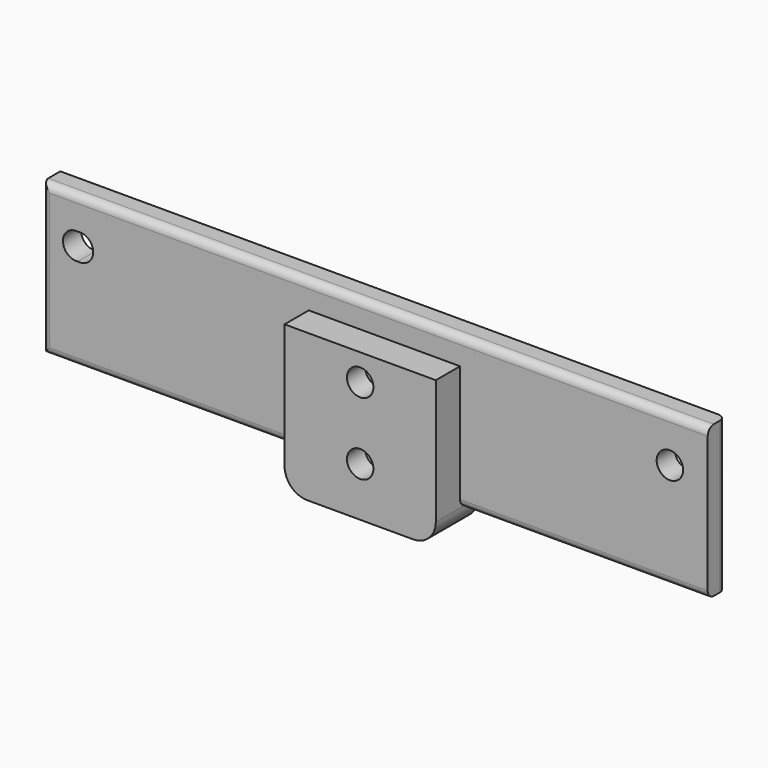
from build123d import *

# Parameters (mm, degrees)
F0_W     = 88
F0_H     = 20
F0_R     = 1.75
F1_DEPTH = 3
F2_W     = 20
F2_H     = 4.5
F2_H_2   = 7.5
F3_DEPTH = 4
F6_DEPTH = 4
F4_R     = 1.75
F7_DEPTH = 25
F9_DEPTH = 3
F10_R    = 3
F11_R    = 1


# Not quite as in the source:
# - a feature names something its author has since deleted; it is built from what else it names


with BuildPart() as f1:
    # F0 (on Front) → F1 (new body)
    with BuildSketch(Plane.XZ):
        with Locations((44, -10)):
            Rectangle(F0_W, F0_H)
        with BuildLine():
            ThreePointArc((35.25, -15.5), (34.0207943633, -16.7498270258), (32.7506918489, -15.5415829716))
            ThreePointArc((32.7506918489, -15.5415829716), (32.75, -15.5), (32.7506918489, -15.4584170284))
            Line((32.7506918489, -15.4584170284), (32.7506918489, -8.0415829716))
            ThreePointArc((32.7506918489, -8.0415829716), (32.75, -8), (32.7506918489, -7.9584170284))
            ThreePointArc((32.7506918489, -7.9584170284), (34.0207943633, -6.7501729742), (35.25, -8))
            Line((35.25, -8), (35.25, -15.5))
        make_face(mode=Mode.SUBTRACT)
        with BuildLine():
            ThreePointArc((4.75, -4.2679491924), (6.1456439237, -4.6771243445), (6.75, -6))
            ThreePointArc((6.75, -6), (6.1456439237, -7.3228756555), (4.75, -7.7320508076))
            ThreePointArc((4.75, -7.7320508076), (2.75, -6), (4.75, -4.2679491924))
        make_face(mode=Mode.SUBTRACT)
        with Locations((83, -6)):
            Circle(F0_R, mode=Mode.SUBTRACT)
    extrude(amount=F1_DEPTH)

    # F2 (on face) → F3 (join)
    with BuildSketch(Plane.XZ.offset(3)):
        with Locations((45.25, -5.75)):
            Rectangle(F2_W, F2_H)
        with Locations((45.25, -11.75)):
            Rectangle(F2_W, F2_H_2)
        with Locations((45.25, -17.75)):
            Rectangle(F2_W, F2_H)
    extrude(amount=F3_DEPTH)

    # F5 (on face) → F6 (cut)
    with BuildSketch(Plane(origin=(0, 0, 0), x_dir=(-1, 0, 0), z_dir=(0, 1, 0))):
        Polygon((-43.5179491924, -4), (-46.9820508076, -4), (-48.7141016151, -7), (-46.9820508076, -10), (-43.5179491924, -10), (-41.7858983849, -7), align=None)
        Polygon((-43.5179491924, -13.5), (-46.9820508076, -13.5), (-48.7141016151, -16.5), (-46.9820508076, -19.5), (-43.5179491924, -19.5), (-41.7858983849, -16.5), align=None)
    extrude(amount=-F6_DEPTH, mode=Mode.SUBTRACT)

    # F4 (on face) → F7 (cut)
    with BuildSketch(Plane.XZ.offset(7)):
        with Locations((45.25, -7)):
            Circle(F4_R)
        with Locations((45.25, -16.5)):
            Circle(F4_R)
    extrude(amount=-F7_DEPTH, mode=Mode.SUBTRACT)

    # F8 (on face) → F9 (join)
    with BuildSketch(Plane(origin=(0, 0, -20), x_dir=(1, 0, 0), z_dir=(0, 0, -1))):
        Polygon((55.25, 3), (55.25, 7), (35.25, 7), (35.25, 3), (35.25, 0), (55.25, 0), align=None)
    extrude(amount=F9_DEPTH)

    # F10
    f10_edges = [f1.edges().sort_by_distance(p)[0] for p in [
        (35.25, -3.5, -23),
        (55.25, -3.5, -23),
    ]]
    fillet(f10_edges, radius=F10_R)

    # F11
    f11_edges = [f1.edges().sort_by_distance(p)[0] for p in [
        (44, -3, 0),
        (88, 0, -10),
        (71.625, -3, -20),
        (17.625, -3, -20),
        (0, -3, -10),
    ]]
    fillet(f11_edges, radius=F11_R)


solid = f1.part
